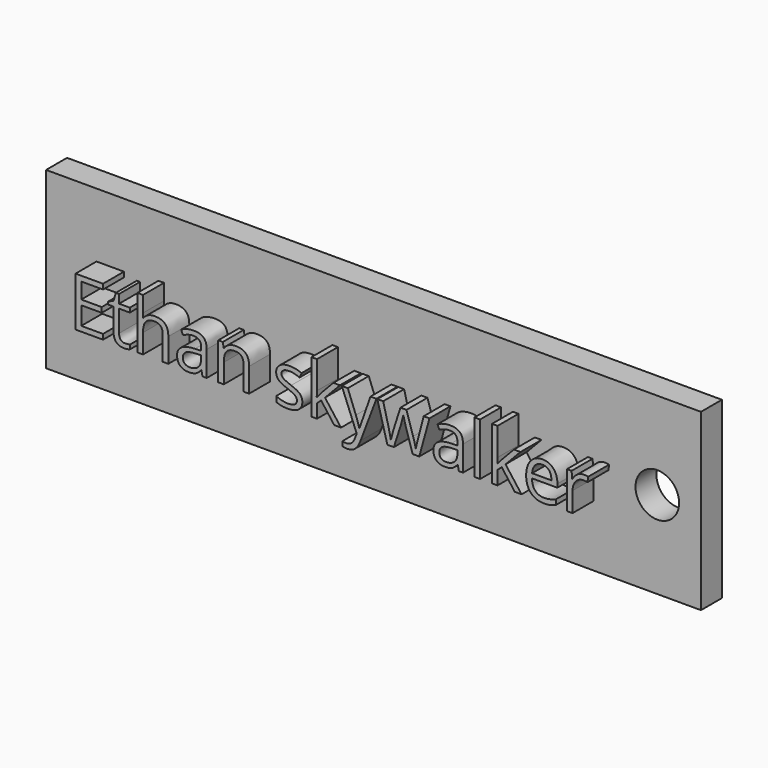
from build123d import *

# Parameters (mm, degrees)
F0_W         = 75
F0_H         = 20
F0_R         = 2.5
F1_DEPTH     = 3
F2_TEXT_SIZE = 7.9051383399
F3_DEPTH     = 3


# Not quite as in the source:
# - Text() gives the source's letters only with a copy of the font that has no kerning and outlines rounded to 1/6400 em; it was checked with that copy


with BuildPart() as f1:
    # F0 (on Front) → F1 (new body)
    with BuildSketch(Plane.XZ):
        with Locations((37.5, -10)):
            Rectangle(F0_W, F0_H)
        with Locations((70, -10)):
            Circle(F0_R, mode=Mode.SUBTRACT)
    extrude(amount=F1_DEPTH)

    # F2 (on face) → F3 (join)
    with BuildSketch(Plane.XZ.offset(3)):
        with Locations((5, -13)):
            Text('Ethan skywalker', F2_TEXT_SIZE, font='Open Sans', text_align=(TextAlign.LEFT, TextAlign.BOTTOM))
    extrude(amount=F3_DEPTH)


solid = f1.part
